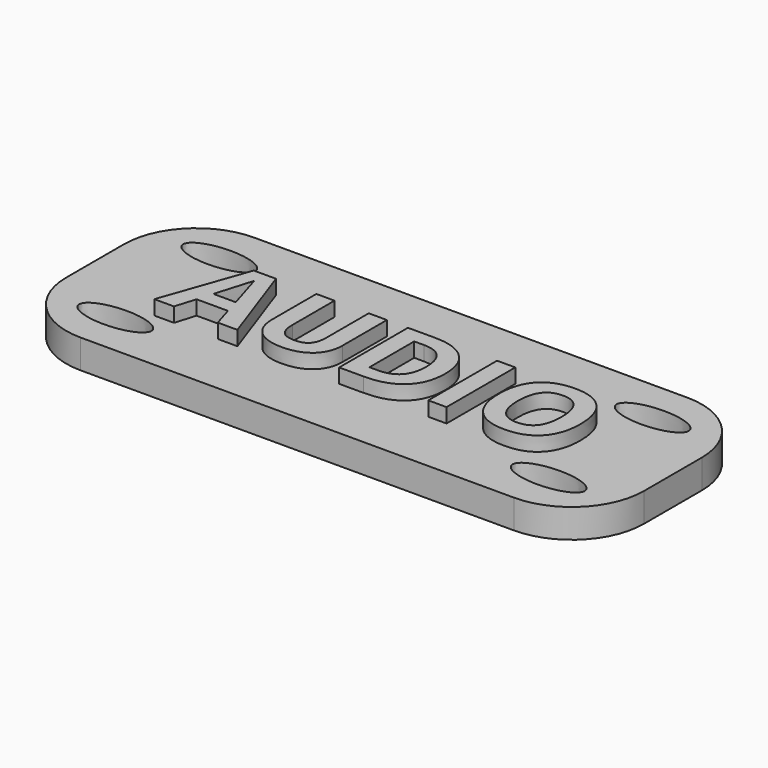
from build123d import *

# Parameters (mm, degrees)
F0_W         = 40
F0_H         = 15
F1_DEPTH     = 2
F2_TEXT_SIZE = 8.3333333333
F3_DEPTH     = 1
F4_R         = 5


# Not quite as in the source:
# - Text() gives the source's letters only with a copy of the font that has no kerning and outlines rounded to 1/6400 em; it was checked with that copy


with BuildPart() as f1:
    # F0 (on Top) → F1 (new body)
    with BuildSketch(Plane.XY):
        Rectangle(F0_W, F0_H)
        with BuildLine():
            add(Edge.make_bspline(
                [(-12.5, -4.5), (-12.5, -2.7679491924), (-16.25, -3.6339745962), (-20, -4.5), (-16.25, -5.3660254038), (-12.5, -6.2320508076), (-12.5, -4.5)],
                knots=[0, 0, 0, 2.0943951024, 2.0943951024, 4.1887902048, 4.1887902048, 6.2831853072, 6.2831853072, 6.2831853072], degree=2, weights=[1, 0.5, 1, 0.5, 1, 0.5, 1]))
        make_face(mode=Mode.SUBTRACT)
        with BuildLine():
            add(Edge.make_bspline(
                [(17.5, -4.5), (17.5, -2.7679491924), (13.75, -3.6339745962), (10, -4.5), (13.75, -5.3660254038), (17.5, -6.2320508076), (17.5, -4.5)],
                knots=[0, 0, 0, 2.0943951024, 2.0943951024, 4.1887902048, 4.1887902048, 6.2831853072, 6.2831853072, 6.2831853072], degree=2, weights=[1, 0.5, 1, 0.5, 1, 0.5, 1]))
        make_face(mode=Mode.SUBTRACT)
        with BuildLine():
            add(Edge.make_bspline(
                [(-12.5, 4.5), (-12.5, 6.2320508076), (-16.25, 5.3660254038), (-20, 4.5), (-16.25, 3.6339745962), (-12.5, 2.7679491924), (-12.5, 4.5)],
                knots=[0, 0, 0, 2.0943951024, 2.0943951024, 4.1887902048, 4.1887902048, 6.2831853072, 6.2831853072, 6.2831853072], degree=2, weights=[1, 0.5, 1, 0.5, 1, 0.5, 1]))
        make_face(mode=Mode.SUBTRACT)
        with BuildLine():
            add(Edge.make_bspline(
                [(17.5, 4.5), (17.5, 6.2320508076), (13.75, 5.3660254038), (10, 4.5), (13.75, 3.6339745962), (17.5, 2.7679491924), (17.5, 4.5)],
                knots=[0, 0, 0, 2.0943951024, 2.0943951024, 4.1887902048, 4.1887902048, 6.2831853072, 6.2831853072, 6.2831853072], degree=2, weights=[1, 0.5, 1, 0.5, 1, 0.5, 1]))
        make_face(mode=Mode.SUBTRACT)
    extrude(amount=F1_DEPTH)

    # F4
    f4_edges = [f1.edges().sort_by_distance(p)[0] for p in [
        (-20, -7.5, 1),
        (20, -7.5, 1),
        (20, 7.5, 1),
        (-20, 7.5, 1),
    ]]
    fillet(f4_edges, radius=F4_R)


with BuildPart() as f3:
    # F2 (on face) → F3 (new body)
    with BuildSketch(Plane.XY.offset(2)):
        with Locations((-13.5, -3)):
            Text('AUDIO', F2_TEXT_SIZE, font='Open Sans', font_style=FontStyle.BOLD, text_align=(TextAlign.LEFT, TextAlign.BOTTOM))
    extrude(amount=F3_DEPTH)


solid = Compound([f1.part, f3.part])
